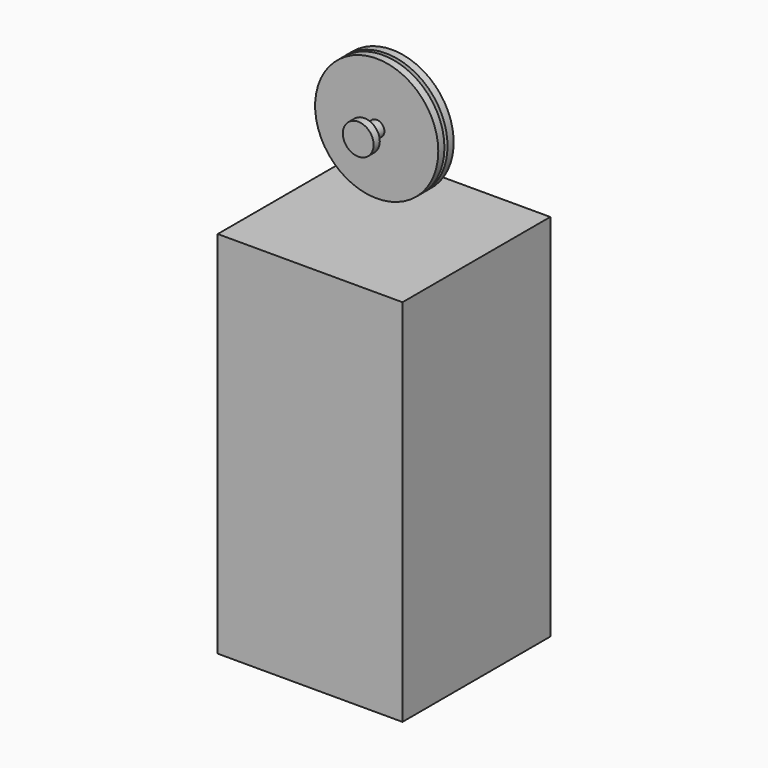
from build123d import *

# Parameters (mm, degrees)
F0_W      = 76.2
F0_H      = 152.4
F1_DEPTH  = 76.2
F3_D      = 50.8
F3_DEPTH  = 127
F3_TIP    = 15.2618597233
F5_R      = 25.4
F7_DEPTH  = 3.175
F8_R      = 3.175
F9_DEPTH  = 1.5875
F10_R     = 3.175
F11_DEPTH = 3.175
F10_R_2   = 25.4
F12_DEPTH = 3.175
F13_R     = 3.175
F14_DEPTH = 6.35
F15_R     = 3.175
F16_DEPTH = 6.35
F17_R     = 3.175
F18_DEPTH = 3.175
F17_R_2   = 6.35
F19_DEPTH = 3.175
F20_R     = 3.175
F21_DEPTH = 3.175
F20_R_2   = 6.35
F22_DEPTH = 3.175


# Not quite as in the source:
# - the program builds the solid bodies; features that only make, move or delete a surface that nothing else refers to are left out


with BuildPart() as f1:
    # F0 (on Front) → F1 (new body)
    with BuildSketch(Plane.XZ):
        with Locations((38.1, 76.2)):
            Rectangle(F0_W, F0_H)
    extrude(amount=-F1_DEPTH)

    # F3
    with Locations(Plane(origin=(0, 0, 0), x_dir=(1, 0, 0), z_dir=(0, 0, -1))):
        with Locations((38.1, -38.1)):
            Hole(F3_D / 2, depth=F3_DEPTH)
            with Locations((0, 0, -(F3_DEPTH + F3_TIP / 2))):  # 118° drill point
                Cone(0, F3_D / 2, F3_TIP, mode=Mode.SUBTRACT)


with BuildPart() as f7:
    # F5 (on offset) → F7 (new body)
    with BuildSketch(Plane.XZ.offset(-38.1)):
        with Locations((37.628673017, 188.7528598309)):
            Circle(F5_R)
    extrude(amount=F7_DEPTH)

    # F8 (on face) → F9 (join)
    with BuildSketch(Plane(origin=(0, 38.1, 0), x_dir=(-1, 0, 0), z_dir=(0, 1, 0))):
        with Locations((-37.628673017, 188.7528598309)):
            Circle(F8_R)
    extrude(amount=F9_DEPTH)

    # F10 (on face) → F11 (join)
    with BuildSketch(Plane(origin=(0, 39.6875, 0), x_dir=(-1, 0, 0), z_dir=(0, 1, 0))):
        with Locations((-37.628673017, 188.7528598309)):
            Circle(F10_R)
    extrude(amount=F11_DEPTH)

    # F10 (on face) → F12 (join)
    with BuildSketch(Plane(origin=(0, 39.6875, 0), x_dir=(-1, 0, 0), z_dir=(0, 1, 0))):
        with Locations((-37.628673017, 188.7528598309)):
            Circle(F10_R_2)
        with Locations((-37.628673017, 188.7528598309)):
            Circle(F10_R, mode=Mode.SUBTRACT)
    extrude(amount=F12_DEPTH)

    # F13 (on face) → F14 (join)
    with BuildSketch(Plane(origin=(0, 42.8625, 0), x_dir=(-1, 0, 0), z_dir=(0, 1, 0))):
        with Locations((-37.628673017, 188.7528598309)):
            Circle(F13_R)
    extrude(amount=F14_DEPTH)

    # F15 (on face) → F16 (join)
    with BuildSketch(Plane.XZ.offset(-34.925)):
        with Locations((37.628673017, 188.7528598309)):
            Circle(F15_R)
    extrude(amount=F16_DEPTH)

    # F17 (on face) → F18 (join)
    with BuildSketch(Plane.XZ.offset(-28.575)):
        with Locations((37.628673017, 188.7528598309)):
            Circle(F17_R)
    extrude(amount=F18_DEPTH)

    # F17 (on face) → F19 (join)
    with BuildSketch(Plane.XZ.offset(-28.575)):
        with Locations((37.628673017, 188.7528598309)):
            Circle(F17_R_2)
        with Locations((37.628673017, 188.7528598309)):
            Circle(F17_R, mode=Mode.SUBTRACT)
    extrude(amount=F19_DEPTH)

    # F20 (on face) → F21 (join)
    with BuildSketch(Plane(origin=(0, 49.2125, 0), x_dir=(-1, 0, 0), z_dir=(0, 1, 0))):
        with Locations((-37.628673017, 188.7528598309)):
            Circle(F20_R)
    extrude(amount=F21_DEPTH)

    # F20 (on face) → F22 (join)
    with BuildSketch(Plane(origin=(0, 49.2125, 0), x_dir=(-1, 0, 0), z_dir=(0, 1, 0))):
        with Locations((-37.628673017, 188.7528598309)):
            Circle(F20_R_2)
    extrude(amount=F22_DEPTH)


solid = Compound([f1.part, f7.part])
